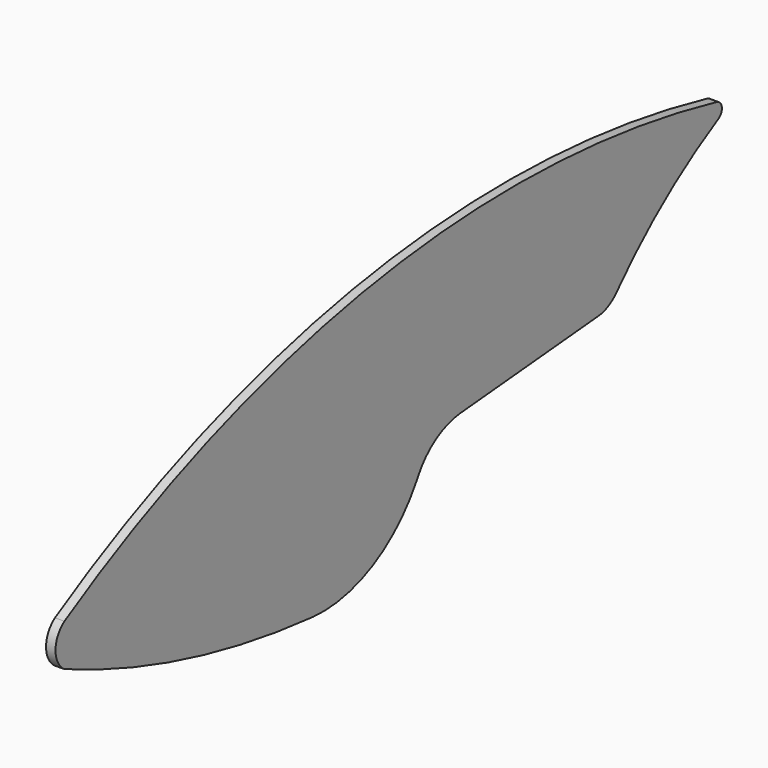
from build123d import *

# Parameters (mm, degrees)
F1_DEPTH = 3.175


# Not quite as in the source:
# - ends of sketch curves that miss each other by under 0.0002 mm in the source are joined


with BuildPart() as f1:
    # F0 (on Right) → F1 (new body)
    with BuildSketch(Plane.YZ):
        with BuildLine():
            ThreePointArc((95.7616986955, -2.4384445977), (115.8206686741, 16.458433146), (138.7853580017, 31.6925169435))
            ThreePointArc((138.7853580017, 31.6925169435), (140.2492541442, 34.5947643313), (138.0609974389, 36.9984236581))
            ThreePointArc((138.0609974389, 36.9984236581), (-3.331363766, 42.4083585784), (-136.5310363288, -5.3296204889))
            ThreePointArc((-136.5310363288, -5.3296204889), (-140.275599037, -12.4275830619), (-136.5310425411, -19.5255553241))
            ThreePointArc((-136.5310425411, -19.5255553241), (-85.3689517348, -37.3376085714), (-31.987598638, -46.5712291765))
            ThreePointArc((-31.987598638, -46.5712291765), (-6.7583016255, -41.5949042645), (11.8270849627, -23.8223232356))
            Line((11.8270849627, -23.8223232356), (12.4481411913, -22.7466161766))
            ThreePointArc((12.4481411913, -22.7466161766), (19.971713381, -14.8813600309), (30.2742956681, -11.3709138521))
            Line((30.2742956681, -11.3709138521), (88.2365367651, -6.2104608931))
            ThreePointArc((88.2365367651, -6.2104608931), (92.3577760693, -5.0399785829), (95.7616986955, -2.4384445977))
        make_face()
    extrude(amount=F1_DEPTH)


solid = f1.part
